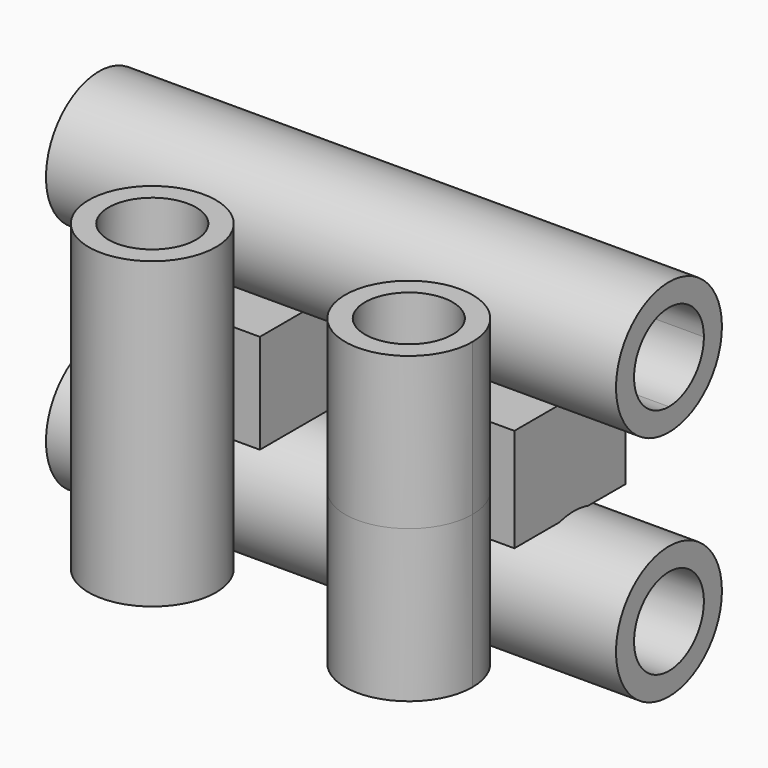
from build123d import *

# Parameters (mm, degrees)
F2_R          = 8.8480516112
F3_DEPTH      = 38.1
F3_DEPTH_BACK = 38.1
F2_R_2        = 5.8358111442
F4_R          = 8.5101971468
F4_R_2        = 5.8539450754
F5_DEPTH      = 20.32
F5_DEPTH_BACK = 20.32
F6_W          = 16.4804635569
F6_H          = 13.8223250397
F7_DEPTH      = 17.78
F7_DEPTH_BACK = 0.762
F6_W_2        = 17.0120932162
F6_H_2        = 13.2906967774


# Not quite as in the source:
# - the program builds the solid bodies; features that only make, move or delete a surface that nothing else refers to are left out


with BuildPart() as f3:
    # F2 (on Right) → F3 (new body, two sides)
    with BuildSketch(Plane.YZ) as f3_sk:
        with Locations((-7.8415106982, 15.5501165427)):
            Circle(F2_R)
        with BuildLine():
            ThreePointArc((-7.8415106982, 21.3859276869), (-3.7149690644, 19.6766581765), (-2.005699554, 15.5501165427))
            ThreePointArc((-2.005699554, 15.5501165427), (-3.7149690644, 11.4235749089), (-7.8415106982, 9.7143053985))
            ThreePointArc((-7.8415106982, 9.7143053985), (-13.6773218424, 15.5501165427), (-7.8415106982, 21.3859276869))
        make_face(mode=Mode.SUBTRACT)
    extrude(amount=F3_DEPTH)
    extrude(f3_sk.sketch, amount=-F3_DEPTH_BACK)


with BuildPart() as f3b:
    # F2 (on Right) → F3, piece 2 (new body, two sides)
    with BuildSketch(Plane.YZ) as f3_2_sk:
        with Locations((-7.8415106982, -15.5501165427)):
            Circle(F2_R)
        with Locations((-7.8415106982, -15.5501165427)):
            Circle(F2_R_2, mode=Mode.SUBTRACT)
    extrude(amount=F3_DEPTH)
    extrude(f3_2_sk.sketch, amount=-F3_DEPTH_BACK)


with BuildPart() as f5:
    # F4 (on Top) → F5 (new body, two sides)
    with BuildSketch(Plane.XY) as f5_sk:
        with Locations((-17.1450003982, -25.1194182783)):
            Circle(F4_R)
        with Locations((-17.1450003982, -25.1194182783)):
            Circle(F4_R_2, mode=Mode.SUBTRACT)
    extrude(amount=F5_DEPTH)
    extrude(f5_sk.sketch, amount=-F5_DEPTH_BACK)


with BuildPart() as f5b:
    # F4 (on Top) → F5, piece 2 (new body, two sides)
    with BuildSketch(Plane.XY) as f5_2_sk:
        with BuildLine():
            ThreePointArc((14.2210470513, -17.1273001421), (12.2695498524, -32.094619885), (25.655197545, -25.1194182783))
            ThreePointArc((25.655197545, -25.1194182783), (22.0204509439, -18.1442166716), (14.2210470513, -17.1273001421))
        make_face()
        with Locations((17.1450003982, -25.1194182783)):
            Circle(F4_R_2, mode=Mode.SUBTRACT)
    extrude(amount=F5_DEPTH)
    extrude(f5_2_sk.sketch, amount=-F5_DEPTH_BACK)


with BuildPart() as f7:
    # F6 (on Front) → F7 (new body, two sides)
    with BuildSketch(Plane.XZ) as f7_sk:
        with Locations((17.1449990012, -0.1329074148)):
            Rectangle(F6_W, F6_H)
    extrude(amount=F7_DEPTH)
    extrude(f7_sk.sketch, amount=-F7_DEPTH_BACK)


with BuildPart() as f7b:
    # F6 (on Front) → F7, piece 2 (new body, two sides)
    with BuildSketch(Plane.XZ) as f7_2_sk:
        with Locations((-17.1450003982, 0.1329067163)):
            Rectangle(F6_W_2, F6_H_2)
    extrude(amount=F7_DEPTH)
    extrude(f7_2_sk.sketch, amount=-F7_DEPTH_BACK)


solid = Compound([f3.part, f3b.part, f5.part, f5b.part, f7.part, f7b.part])
